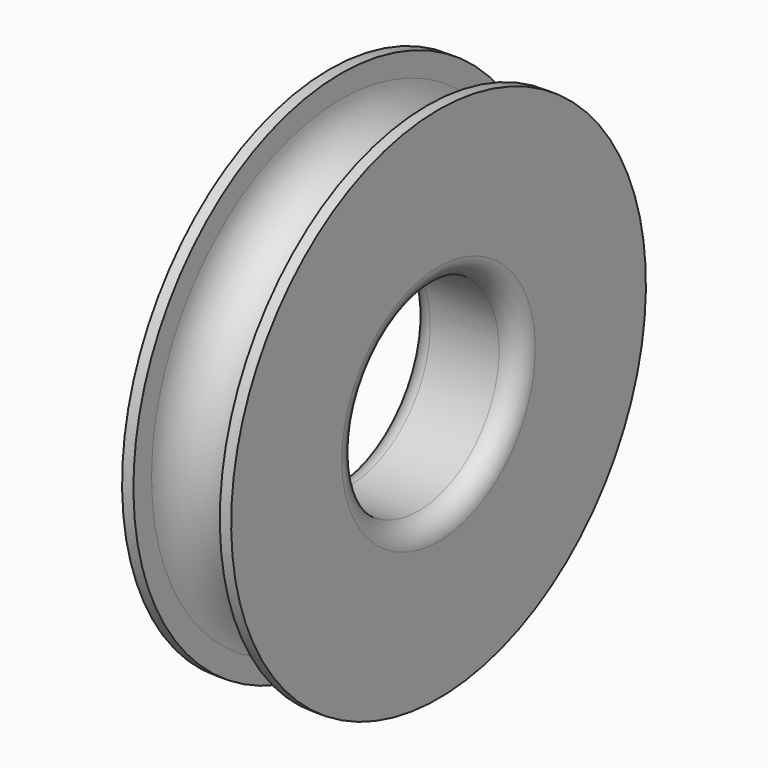
from build123d import *

# Parameters (mm, degrees)
F3_R     = 8.89
F4_DEPTH = 25.4
F5_R     = 1.778


with BuildPart() as f2:
    # F0 (on Front) → F2 (revolve)
    with BuildSketch(Plane.XZ):
        with BuildLine():
            Line((-3.81, 0), (0, 0))
            Line((0, 0), (3.81, 0))
            Line((3.81, 0), (3.81, 20.86))
            ThreePointArc((3.81, 20.86), (0, 17.05), (-3.81, 20.86))
            Line((-3.81, 20.86), (-3.81, 0))
        make_face()
        Polygon((-4.81, 0), (-3.81, 0), (-3.81, 20.86), (-3.81, 22.86), (-4.81, 22.86), align=None)
        Polygon((3.81, 20.86), (3.81, 0), (4.81, 0), (4.81, 22.86), (3.81, 22.86), align=None)
    revolve(axis=Axis((-0.3435998224, 0, 0), (1, 0, 0)))

    # F3 (on face) → F4 (cut)
    with BuildSketch(Plane(origin=(-4.81, 0, 0), x_dir=(0, -1, 0), z_dir=(-1, 0, 0))):
        Circle(F3_R)
    extrude(amount=-F4_DEPTH, mode=Mode.SUBTRACT)

    # F5
    f5_edges = [f2.edges().sort_by_distance(p)[0] for p in [
        (4.81, 8.89, 0),
        (-4.81, 8.89, 0),
    ]]
    fillet(f5_edges, radius=F5_R)


solid = f2.part
